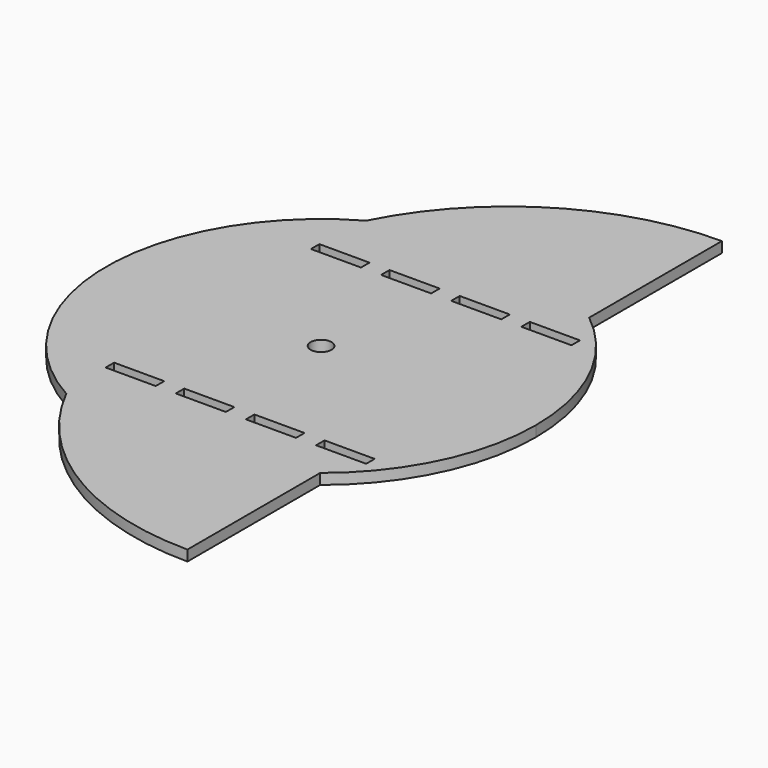
from build123d import *

# Parameters (mm, degrees)
F0_R     = 3.125
F1_DEPTH = 3.175
F2_W     = 15
F2_H     = 3.175
F2_W_2   = 7.5
F3_DEPTH = 25


# Not quite as in the source:
# - a feature names something its author has since deleted; it is built from what else it names


with BuildPart() as f1:
    # F0 (on Top) → F1 (new body)
    with BuildSketch(Plane.XY):
        with BuildLine():
            ThreePointArc((40, -50.3277523465), (57.898111611, -27.9408541051), (64.2875, 0))
            ThreePointArc((64.2875, 0), (57.898111611, 27.9408541051), (40, 50.3277523465))
            Line((40, 50.3277523465), (40, -50.3277523465))
        make_face()
        with BuildLine():
            Line((40, -50.3277523465), (40, 50.3277523465))
            ThreePointArc((40, 50.3277523465), (5.1835564074, 64.0781819282), (-31.390378499, 56.1028234043))
            ThreePointArc((-31.390378499, 56.1028234043), (-37.8178330459, 38.5576092221), (-40, 20))
            Line((-40, 20), (-40, -20))
            ThreePointArc((-40, -20), (-37.8178330459, -38.5576092221), (-31.390378499, -56.1028234043))
            ThreePointArc((-31.390378499, -56.1028234043), (5.1835564074, -64.0781819282), (40, -50.3277523465))
        make_face()
        Circle(F0_R, mode=Mode.SUBTRACT)
        with BuildLine():
            ThreePointArc((-31.390378499, 56.1028234043), (5.1835564074, 64.0781819282), (40, 50.3277523465))
            Line((40, 50.3277523465), (40, 100))
            ThreePointArc((40, 100), (-1.9033061205, 88.1477287675), (-31.390378499, 56.1028234043))
        make_face()
        with BuildLine():
            Line((40, -100), (40, -50.3277523465))
            ThreePointArc((40, -50.3277523465), (5.1835564074, -64.0781819282), (-31.390378499, -56.1028234043))
            ThreePointArc((-31.390378499, -56.1028234043), (-1.9033061205, -88.1477287675), (40, -100))
        make_face()
        with BuildLine():
            ThreePointArc((-40, 20), (-37.8178330459, 38.5576092221), (-31.390378499, 56.1028234043))
            ThreePointArc((-31.390378499, 56.1028234043), (-64.2875, 0), (-31.390378499, -56.1028234043))
            ThreePointArc((-31.390378499, -56.1028234043), (-37.8178330459, -38.5576092221), (-40, -20))
            Line((-40, -20), (-40, 20))
        make_face()
    extrude(amount=F1_DEPTH)

    # F2 (on face) → F3 (cut)
    with BuildSketch(Plane.XY.offset(3.175)):
        with Locations((-4, 38.4125)):
            Rectangle(F2_W, F2_H)
        with Locations((13.25, 38.4125)):
            Rectangle(F2_W_2, F2_H)
        with Locations((20.75, 38.4125)):
            Rectangle(F2_W_2, F2_H)
        with Locations((38, 38.4125)):
            Rectangle(F2_W, F2_H)
        with Locations((-4, -38.4125)):
            Rectangle(F2_W, F2_H)
        with Locations((20.75, -38.4125)):
            Rectangle(F2_W_2, F2_H)
        with Locations((38, -38.4125)):
            Rectangle(F2_W, F2_H)
        with Locations((13.25, -38.4125)):
            Rectangle(F2_W_2, F2_H)
        with Locations((-25, -38.4125)):
            Rectangle(F2_W, F2_H)
        with Locations((-25, 38.4125)):
            Rectangle(F2_W, F2_H)
    extrude(amount=-F3_DEPTH, mode=Mode.SUBTRACT)


solid = f1.part
